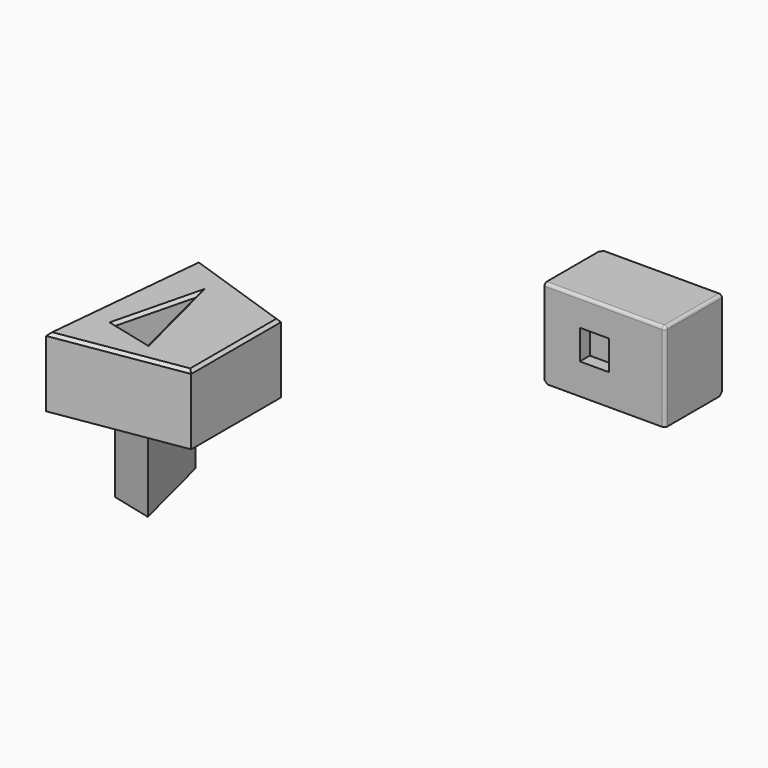
from build123d import *

# Parameters (mm, degrees)
F0_W      = 207.5331061672
F0_H      = 122.6332091976
F1_DEPTH  = 152.4
F3_DEPTH  = 144.78
F4_DEPTH  = 119.38
F5_R      = 5.08
F6_SIZE   = 5.08
F7_SIZE   = 5.08
F8_R      = 30.0636447878
F9_DEPTH  = 11.684
F10_W     = 50.5407005548
F10_H     = 51.1219091713
F11_DEPTH = 21.59


# Not quite as in the source:
# - the program builds the solid bodies; features that only make, move or delete a surface that nothing else refers to are left out


with BuildPart() as f1:
    # F0 (on Top) → F1 (new body)
    with BuildSketch(Plane.XY):
        with Locations((212.2609269613, 171.3262020208)):
            Rectangle(F0_W, F0_H)
    extrude(amount=F1_DEPTH)

    # F5
    f5_edges = [f1.edges().sort_by_distance(p)[0] for p in [
        (212.260927, 110.009597, 152.4),
        (316.02748, 171.326202, 152.4),
        (316.02748, 110.009597, 76.2),
    ]]
    fillet(f5_edges, radius=F5_R)

    # F6
    f6_edges = [f1.edges().sort_by_distance(p)[0] for p in [
        (108.494374, 232.642807, 76.2),
        (212.260927, 232.642807, 0),
        (108.494374, 171.326202, 0),
    ]]
    chamfer(f6_edges, length=F6_SIZE)

    # F8 (on face) → F9 (join)
    with BuildSketch(Plane(origin=(0, 232.6428066196, 0), x_dir=(-1, 0, 0), z_dir=(0, 1, 0))):
        with Locations((-219.7953462601, 82.3513418436)):
            Circle(F8_R)
    extrude(amount=F9_DEPTH)

    # F10 (on face) → F11 (cut)
    with BuildSketch(Plane.XZ.offset(-110.009597422)):
        with Locations((194.4875046611, 78.6354225129)):
            Rectangle(F10_W, F10_H)
    extrude(amount=-F11_DEPTH, mode=Mode.SUBTRACT)


with BuildPart() as f3:
    # F0 (on Top) → F3 (new body)
    with BuildSketch(Plane.XY):
        Polygon((-238.994547933, -309.9301279931), (-277.0052831988, -160.1067611335), (-310.0219274309, -292.1732745837), align=None)
    extrude(amount=-F3_DEPTH)


with BuildPart() as f4:
    # F0 (on Top) → F4 (new body)
    with BuildSketch(Plane.XY):
        Polygon((-142.5804198811, -143.5984707565), (-335.9635537997, -77.565192872), (-364.2635406156, -372.3565564559), (-142.5804198811, -336.9815940954), align=None)
        Polygon((-310.0219274309, -292.1732745837), (-277.0052831988, -160.1067611335), (-238.994547933, -309.9301279931), align=None, mode=Mode.SUBTRACT)
    extrude(amount=F4_DEPTH)

    # F7
    f7_edges = [f4.edges().sort_by_distance(p)[0] for p in [
        (-350.113547, -224.960875, 119.38),
        (-253.42198, -354.669075, 119.38),
        (-142.58042, -240.290032, 119.38),
        (-239.271987, -110.581832, 119.38),
        (-274.508238, -301.051701, 119.38),
        (-293.513605, -226.140018, 119.38),
        (-257.999916, -235.018445, 119.38),
    ]]
    chamfer(f7_edges, length=F7_SIZE)


solid = Compound([f1.part, f3.part, f4.part])
